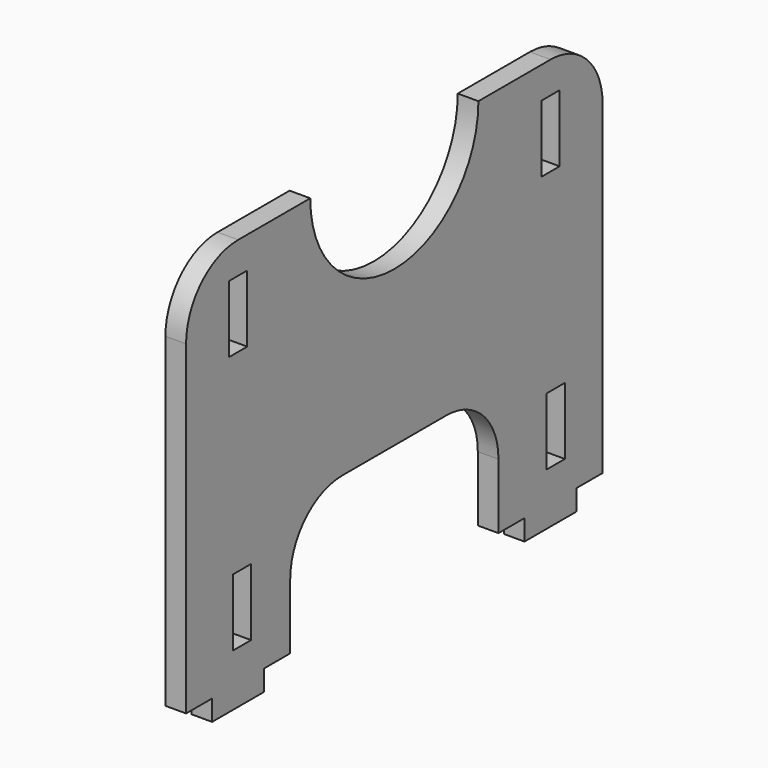
from build123d import *

# Parameters (mm, degrees)
F0_W     = 1.74625
F0_H     = 5.15
F0_W_2   = 5
F0_H_2   = 1.5875
F1_DEPTH = 1.5875
F2_R     = 5


# Not quite as in the source:
# - a length typed as a fraction of an inch, garbled in the dataset ("3 / 203.2 mm" for 3/8 in), is restored


with BuildPart() as f1:
    # F0 (on Right) → F1 (new body)
    with BuildSketch(Plane.YZ):
        with BuildLine():
            Line((20, -15), (20, 15))
            Line((20, 15), (8.075, 15))
            ThreePointArc((8.075, 15), (0, 6.925), (-8.075, 15))
            Line((-8.075, 15), (-20, 15))
            Line((-20, 15), (-20, -15))
            Line((-20, -15), (-17.5, -15))
            Line((-17.5, -15), (-12.5, -15))
            Line((-12.5, -15), (-10, -15))
            Line((-10, -15), (-10, -5))
            Line((-10, -5), (10, -5))
            Line((10, -5), (10, -15))
            Line((10, -15), (12.5, -15))
            Line((12.5, -15), (17.5, -15))
            Line((17.5, -15), (20, -15))
        make_face()
        with Locations((-14.6303550991, -10)):
            Rectangle(F0_W, F0_H, mode=Mode.SUBTRACT)
        with Locations((15.5080378336, -10)):
            Rectangle(F0_W, F0_H, mode=Mode.SUBTRACT)
        with Locations((-15, 10)):
            Rectangle(F0_W, F0_H, mode=Mode.SUBTRACT)
        with Locations((15, 10)):
            Rectangle(F0_W, F0_H, mode=Mode.SUBTRACT)
        with Locations((-15, -15.79375)):
            Rectangle(F0_W_2, F0_H_2)
        with Locations((15, -15.79375)):
            Rectangle(F0_W_2, F0_H_2)
    extrude(amount=F1_DEPTH)

    # F2
    f2_edges = [f1.edges().sort_by_distance(p)[0] for p in [
        (0.79375, -10, -5),
        (0.79375, 10, -5),
        (0.79375, 20, 15),
        (0.79375, -20, 15),
    ]]
    fillet(f2_edges, radius=F2_R)


solid = f1.part
